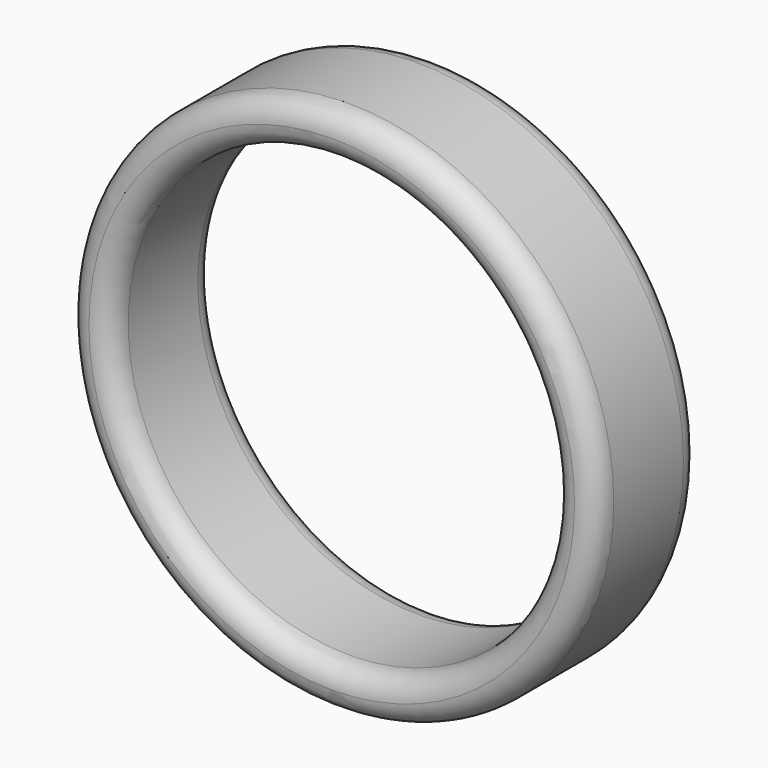
from build123d import *

# Parameters (mm, degrees)
F0_R     = 12.15
F0_R_2   = 10.15
F1_DEPTH = 6
F2_R     = 1
F3_R     = 0.99999


# Not quite as in the source:
# - a fillet or chamfer is up to 0.001 mm smaller than in the source, because OpenCascade refuses the exact size


with BuildPart() as f1:
    # F0 (on Front) → F1 (new body)
    with BuildSketch(Plane.XZ):
        Circle(F0_R)
        Circle(F0_R_2, mode=Mode.SUBTRACT)
    extrude(amount=F1_DEPTH)

    # F2
    f2_edges = [f1.edges().sort_by_distance(p)[0] for p in [
        (-10.15, -6, 0),
        (-10.15, 0, 0),
    ]]
    fillet(f2_edges, radius=F2_R)

    # F3 (radius 1 in the source; OpenCascade refuses exactly that, so slightly less here)
    f3_edges = [f1.edges().sort_by_distance(p)[0] for p in [
        (-12.15, 0, 0),
        (-12.15, -6, 0),
    ]]
    fillet(f3_edges, radius=F3_R)


solid = f1.part
